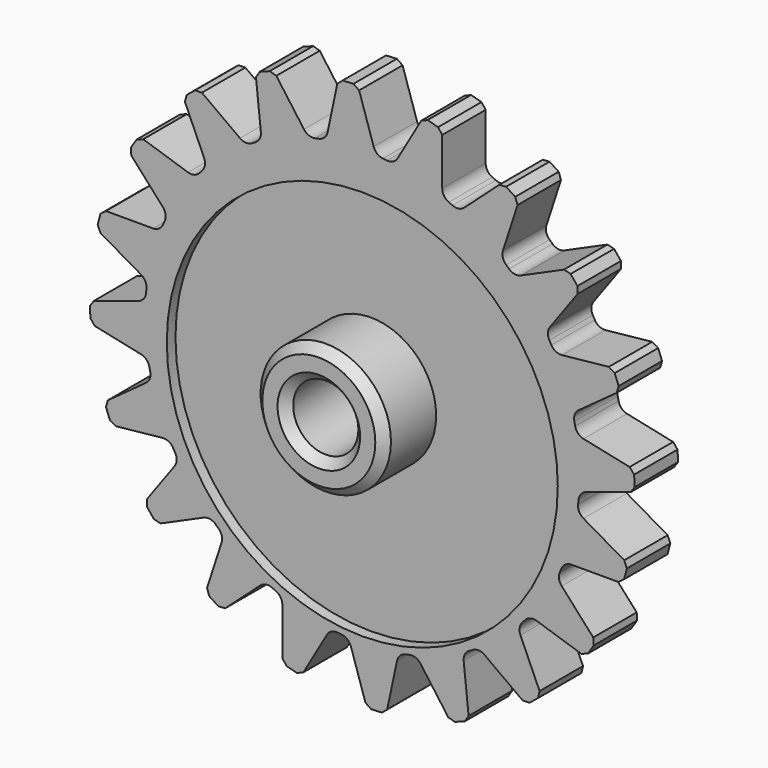
from build123d import *

# Parameters (mm, degrees)
F0_R            = 100
F1_DEPTH        = 25
F3_DEPTH        = 25
F3_COPIES_COUNT = 20
F4_R            = 5
F5_SIZE         = 2
F6_R            = 90
F7_DEPTH        = 5
F8_R            = 30
F9_DEPTH        = 30
F10_R           = 15
F11_DEPTH       = 50.001
F12_SIZE        = 4


# Not quite as in the source:
# - a pattern or mirror of a feature is missing from the dataset's text; its kind, count and spacing are read off the source's solid


with BuildPart() as f1:
    # F0 (on Front) → F1 (new body)
    with BuildSketch(Plane.XZ):
        Circle(F0_R)
    extrude(amount=F1_DEPTH)

    # F2 (on face) → F3 (join)
    with BuildSketch(Plane.XZ.offset(25)):
        Polygon((28.119313467, 122.3293714059), (14.6081000224, 98.927263248), (36.8126459036, 92.9775731108), (36.8126459036, 120), align=None)
    f3 = extrude(amount=-F3_DEPTH)

    # F3_copies: F3 ×20 about axis
    f3_copies_axis = Axis((0, 0, 0), (0, 1, 0))
    for i in range(1, F3_COPIES_COUNT):
        add(f3.rotate(f3_copies_axis, i * 360 / F3_COPIES_COUNT))

    # F4
    f4_edges = [f1.edges().sort_by_distance(p)[0] for p in [
        (14.6081, -12.5, 98.927263),
        (36.812646, -12.5, 92.977573),
        (6.279257, -12.5, 99.80266),
        (99.80266, -12.5, -6.279257),
        (98.927263, -12.5, -14.6081),
        (92.977573, -12.5, -36.812646),
        (89.571267, -12.5, -44.463334),
        (77.051194, -12.5, -63.742557),
        (71.447411, -12.5, -69.966188),
        (53.582506, -12.5, -84.432902),
        (46.329785, -12.5, -88.620263),
        (24.86879, -12.5, -96.858367),
        (16.677077, -12.5, -98.59957),
        (-6.279257, -12.5, -99.80266),
        (-14.6081, -12.5, -98.927263),
        (-36.812646, -12.5, -92.977573),
        (-44.463334, -12.5, -89.571267),
        (-63.742557, -12.5, -77.051194),
        (-69.966188, -12.5, -71.447411),
        (-84.432902, -12.5, -53.582506),
        (-88.620263, -12.5, -46.329785),
        (-96.858367, -12.5, -24.86879),
        (-98.59957, -12.5, -16.677077),
        (-99.80266, -12.5, 6.279257),
        (-98.927263, -12.5, 14.6081),
        (-92.977573, -12.5, 36.812646),
        (-89.571267, -12.5, 44.463334),
        (-77.051194, -12.5, 63.742557),
        (-71.447411, -12.5, 69.966188),
        (-53.582506, -12.5, 84.432902),
        (-46.329785, -12.5, 88.620263),
        (-24.86879, -12.5, 96.858367),
        (-16.677077, -12.5, 98.59957),
        (44.463334, -12.5, 89.571267),
        (63.742557, -12.5, 77.051194),
        (69.966188, -12.5, 71.447411),
        (84.432902, -12.5, 53.582506),
        (88.620263, -12.5, 46.329785),
        (96.858367, -12.5, 24.86879),
        (98.59957, -12.5, 16.677077),
    ]]
    fillet(f4_edges, radius=F4_R)

    # F5
    f5_edges = [f1.edges().sort_by_distance(p)[0] for p in [
        (36.812646, -12.5, 120),
        (28.119313, -12.5, 122.329371),
        (125.502515, -12.5, 2.071133),
        (125.031492, -12.5, 11.058798),
        (122.329371, -12.5, -28.119313),
        (120, -12.5, -36.812646),
        (118.71997, -12.5, 40.752174),
        (115.494658, -12.5, 49.154398),
        (107.6528, -12.5, -64.544911),
        (102.751049, -12.5, -72.092946),
        (100.316286, -12.5, 75.444109),
        (94.652403, -12.5, 82.438423),
        (82.438423, -12.5, -94.652403),
        (75.444109, -12.5, -100.316286),
        (72.092946, -12.5, 102.751049),
        (64.544911, -12.5, 107.6528),
        (49.154398, -12.5, -115.494658),
        (40.752174, -12.5, -118.71997),
        (11.058798, -12.5, -125.031492),
        (2.071133, -12.5, -125.502515),
        (-2.071133, -12.5, 125.502515),
        (-11.058798, -12.5, 125.031492),
        (-28.119313, -12.5, -122.329371),
        (-36.812646, -12.5, -120),
        (-40.752174, -12.5, 118.71997),
        (-49.154398, -12.5, 115.494658),
        (-64.544911, -12.5, -107.6528),
        (-72.092946, -12.5, -102.751049),
        (-75.444109, -12.5, 100.316286),
        (-82.438423, -12.5, 94.652403),
        (-94.652403, -12.5, -82.438423),
        (-100.316286, -12.5, -75.444109),
        (-102.751049, -12.5, 72.092946),
        (-107.6528, -12.5, 64.544911),
        (-115.494658, -12.5, -49.154398),
        (-118.71997, -12.5, -40.752174),
        (-120, -12.5, 36.812646),
        (-122.329371, -12.5, 28.119313),
        (-125.031492, -12.5, -11.058798),
        (-125.502515, -12.5, -2.071133),
    ]]
    chamfer(f5_edges, length=F5_SIZE)

    # F6 (on face) → F7 (cut)
    with BuildSketch(Plane.XZ.offset(25)):
        with Locations((0, -7.1707219706)):
            Circle(F6_R)
    extrude(amount=-F7_DEPTH, mode=Mode.SUBTRACT)

    # F8 (on face) → F9 (join)
    with BuildSketch(Plane.XZ.offset(20)):
        Circle(F8_R)
    extrude(amount=F9_DEPTH)

    # F10 (on face) → F11 (cut, through all)
    with BuildSketch(Plane.XZ.offset(50)):
        Circle(F10_R)
    extrude(amount=-F11_DEPTH, mode=Mode.SUBTRACT)

    # F12
    f12_edges = [f1.edges().sort_by_distance(p)[0] for p in [
        (-30, -50, 0),
        (-15, -50, 0),
    ]]
    chamfer(f12_edges, length=F12_SIZE)


solid = f1.part
